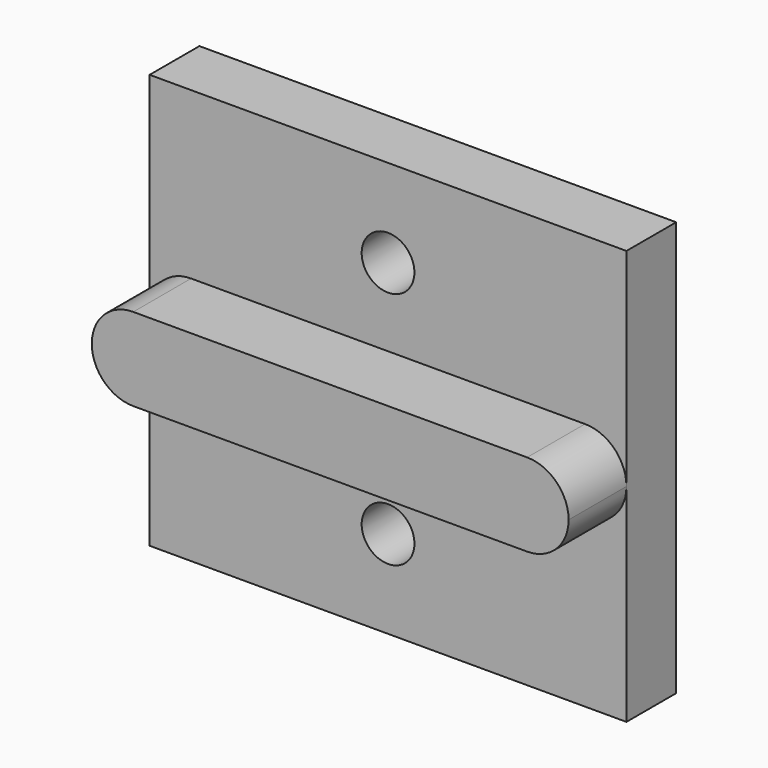
from build123d import *

# Parameters (mm, degrees)
F1_DEPTH = 36.5125
F2_R     = 2.0193
F3_DEPTH = 4.7625
F4_R     = 3.17499


# Not quite as in the source:
# - a fillet or chamfer is up to 0.001 mm smaller than in the source, because OpenCascade refuses the exact size


with BuildPart() as f1:
    # F0 (on Right) → F1 (new body)
    with BuildSketch(Plane.YZ):
        Polygon((-4.7625, 0), (0, 0), (0, 31.75), (-4.7625, 31.75), (-4.7625, 19.05), (-10.2997, 19.05), (-10.2997, 12.7), (-4.7625, 12.7), align=None)
    extrude(amount=-F1_DEPTH)

    # F2 (on face) → F3 (cut, through all)
    with BuildSketch(Plane.XZ.offset(4.7625)):
        with Locations((-18.25625, 25.019)):
            Circle(F2_R)
        with Locations((-18.25625, 6.731)):
            Circle(F2_R)
    extrude(amount=-F3_DEPTH, mode=Mode.SUBTRACT)

    # F4 (radius 3.175 in the source; OpenCascade refuses exactly that, so slightly less here)
    f4_edges = [f1.edges().sort_by_distance(p)[0] for p in [
        (0, -7.5311, 19.05),
        (0, -7.5311, 12.7),
        (-36.5125, -7.5311, 12.7),
        (-36.5125, -7.5311, 19.05),
    ]]
    fillet(f4_edges, radius=F4_R)


solid = f1.part
